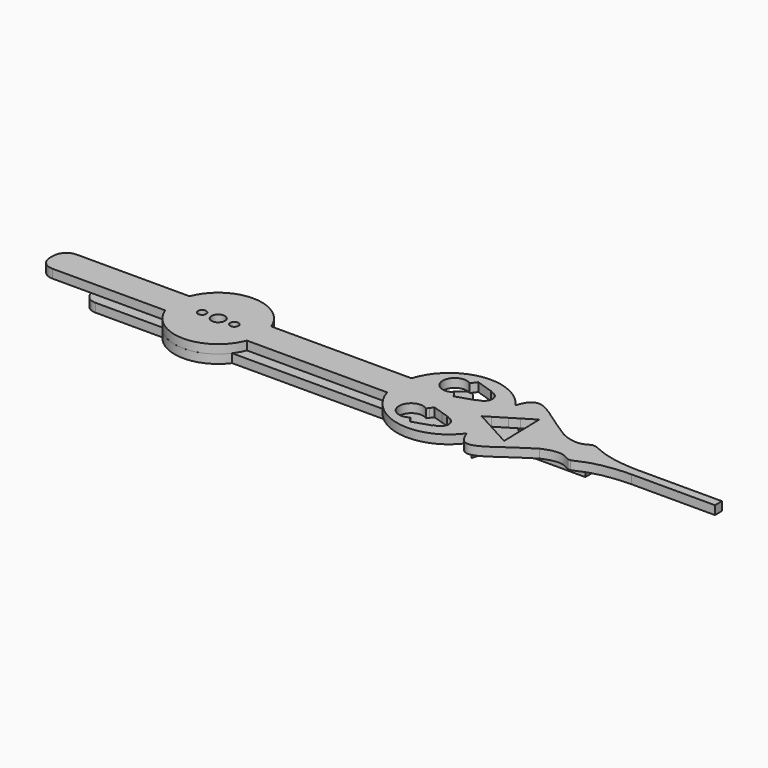
from build123d import *

# Parameters (mm, degrees)
F0_R     = 0.95
F0_R_2   = 1.5375
F1_DEPTH = 2
F2_R     = 0.95
F2_R_2   = 1.7859375
F3_DEPTH = 2
F4_R     = 3
F4_2_R   = 3


with BuildPart() as f1:
    # F0 (on Top) → F1 (new body)
    with BuildSketch(Plane.XY):
        with BuildLine():
            Line((-9.3674969976, 3.5), (-38.25, 3.5))
            Line((-38.25, 3.5), (-38.25, -3.5))
            Line((-38.25, -3.5), (-9.3674969976, -3.5))
            ThreePointArc((-9.3674969976, -3.5), (-10, 0), (-9.3674969976, 3.5))
        make_face()
        with BuildLine():
            ThreePointArc((9.3674969976, 3.5), (0, 10), (-9.3674969976, 3.5))
            Line((-9.3674969976, 3.5), (9.3674969976, 3.5))
        make_face()
        with BuildLine():
            Line((9.3674969976, 3.5), (-9.3674969976, 3.5))
            ThreePointArc((-9.3674969976, 3.5), (-10, 0), (-9.3674969976, -3.5))
            Line((-9.3674969976, -3.5), (9.3674969976, -3.5))
            ThreePointArc((9.3674969976, -3.5), (9.8406038935, -1.7783461452), (10, 0))
            ThreePointArc((10, 0), (9.8406038935, 1.7783461452), (9.3674969976, 3.5))
        make_face()
        with Locations((-3.7, 0)):
            Circle(F0_R, mode=Mode.SUBTRACT)
        Circle(F0_R_2, mode=Mode.SUBTRACT)
        with Locations((3.7, 0)):
            Circle(F0_R, mode=Mode.SUBTRACT)
        with BuildLine():
            Line((41.5486460336, 3.5), (9.3674969976, 3.5))
            ThreePointArc((9.3674969976, 3.5), (9.8406038935, 1.7783461452), (10, 0))
            ThreePointArc((10, 0), (9.8406038935, -1.7783461452), (9.3674969976, -3.5))
            Line((9.3674969976, -3.5), (41.5486460336, -3.5))
            ThreePointArc((41.5486460336, -3.5), (41.0242157381, 0), (41.5486460336, 3.5))
        make_face()
        with BuildLine():
            Line((9.3674969976, -3.5), (-9.3674969976, -3.5))
            ThreePointArc((-9.3674969976, -3.5), (0, -10), (9.3674969976, -3.5))
        make_face()
        with BuildLine():
            ThreePointArc((62.6500663761, 6.9867862956), (51.0189547822, 11.7817934467), (41.5486460336, 3.5))
            Line((41.5486460336, 3.5), (51.2676081814, 3.5))
            Line((51.2676081814, 3.5), (50.8795437488, 4.034124869))
            ThreePointArc((50.8795437488, 4.034124869), (46.4980966164, 6.2665836886), (50.8795437488, 8.4990425082))
            Line((50.8795437488, 8.4990425082), (51.8198733731, 9.7932952023))
            Line((51.8198733731, 9.7932952023), (55.9657714069, 8.4462112726))
            Line((55.9657714069, 8.4462112726), (55.9657714069, 8.2063436542))
            ThreePointArc((55.9657714069, 8.2063436542), (57.3373888325, 7.6382011141), (57.9055313725, 6.2665836886))
            ThreePointArc((57.9055313725, 6.2665836886), (57.3373888325, 4.894966263), (55.9657714069, 4.3268237229))
            Line((55.9657714069, 4.3268237229), (55.9657714069, 4.0869561045))
            Line((55.9657714069, 4.0869561045), (54.1593062669, 3.5))
            Line((54.1593062669, 3.5), (62.0300889952, 3.5))
            add(Edge.make_bspline(
                [(62.6500663761, 6.9867862956), (62.325026984, 5.9395183136), (62.1150441282, 4.7229315023), (62.0300889952, 3.5)],
                knots=[0.7171634713, 0.7171634713, 0.7171634713, 0.7171634713, 0.8591293722, 0.8591293722, 0.8591293722, 0.8591293722], degree=3))
        make_face()
        with BuildLine():
            Line((51.2676081814, 3.5), (41.5486460336, 3.5))
            ThreePointArc((41.5486460336, 3.5), (41.0242157381, 0), (41.5486460336, -3.5))
            Line((41.5486460336, -3.5), (51.2676081814, -3.5))
            Line((51.2676081814, -3.5), (51.8198733731, -2.7398721748))
            Line((51.8198733731, -2.7398721748), (54.1593062669, -3.5))
            Line((54.1593062669, -3.5), (62.0300889952, -3.5))
            add(Edge.make_bspline(
                [(62.0300889952, -3.5), (61.9699977026, -2.634984173), (61.9724597012, -1.7667939996), (62.0410036734, -0.953104062)],
                knots=[0.8591293722, 0.8591293722, 0.8591293722, 0.8591293722, 0.9595460766, 0.9595460766, 0.9595460766, 0.9595460766], degree=3))
            Line((62.0410036734, -0.953104062), (60.5553723025, -0.141462227))
            Line((60.5553723025, -0.141462227), (62.057291222, 0.7735505189))
            add(Edge.make_bspline(
                [(62.0300889952, 3.5), (61.9655550988, 2.5710327675), (61.9731656392, 1.6384044737), (62.057291222, 0.7735505189)],
                knots=[0.8591293722, 0.8591293722, 0.8591293722, 0.8591293722, 0.9669699747, 0.9669699747, 0.9669699747, 0.9669699747], degree=3))
            Line((62.0300889952, 3.5), (54.1593062669, 3.5))
            Line((54.1593062669, 3.5), (51.8198733731, 2.7398721748))
            Line((51.8198733731, 2.7398721748), (51.2676081814, 3.5))
        make_face()
        with BuildLine():
            ThreePointArc((64.3828967802, 3.5), (63.6595501958, 5.3144940497), (62.6500663761, 6.9867862956))
            add(Edge.make_bspline(
                [(62.6500663761, 6.9867862956), (62.325026984, 5.9395183136), (62.1150441282, 4.7229315023), (62.0300889952, 3.5)],
                knots=[0.7171634713, 0.7171634713, 0.7171634713, 0.7171634713, 0.8591293722, 0.8591293722, 0.8591293722, 0.8591293722], degree=3))
            Line((62.0300889952, 3.5), (64.3828967802, 3.5))
        make_face()
        with BuildLine():
            add(Edge.make_bspline(
                [(76.5, 3.5), (70.4279765487, 7.1543273516), (65.4370003335, 12.5197019264), (63.0607100626, 8.3098689603), (62.6500663761, 6.9867862956)],
                knots=[0, 0, 0, 0, 0.5378085921, 0.7171634713, 0.7171634713, 0.7171634713, 0.7171634713], degree=3))
            ThreePointArc((62.6500663761, 6.9867862956), (63.6595501958, 5.3144940497), (64.3828967802, 3.5))
            Line((64.3828967802, 3.5), (66.5325360501, 3.5))
            Line((66.5325360501, 3.5), (69.4303606274, 5.2654391254))
            Line((69.4303606274, 5.2654391254), (69.4719960261, 3.5))
            Line((69.4719960261, 3.5), (76.5, 3.5))
        make_face()
        with BuildLine():
            Line((51.2676081814, -3.5), (41.5486460336, -3.5))
            ThreePointArc((41.5486460336, -3.5), (51.0189547822, -11.7817934467), (62.6500663761, -6.9867862956))
            add(Edge.make_bspline(
                [(62.6500663761, -6.9867862956), (62.325026984, -5.9395183136), (62.1150441282, -4.7229315023), (62.0300889952, -3.5)],
                knots=[0.7171634713, 0.7171634713, 0.7171634713, 0.7171634713, 0.8591293722, 0.8591293722, 0.8591293722, 0.8591293722], degree=3))
            Line((62.0300889952, -3.5), (54.1593062669, -3.5))
            Line((54.1593062669, -3.5), (55.9657714069, -4.0869561045))
            Line((55.9657714069, -4.0869561045), (55.9657714069, -4.3268237229))
            ThreePointArc((55.9657714069, -4.3268237229), (57.3373888325, -4.894966263), (57.9055313725, -6.2665836886))
            ThreePointArc((57.9055313725, -6.2665836886), (57.3373888325, -7.6382011141), (55.9657714069, -8.2063436542))
            Line((55.9657714069, -8.2063436542), (55.9657714069, -8.4462112726))
            Line((55.9657714069, -8.4462112726), (51.8198733731, -9.7932952023))
            Line((51.8198733731, -9.7932952023), (50.8795437488, -8.4990425082))
            ThreePointArc((50.8795437488, -8.4990425082), (46.4980966164, -6.2665836886), (50.8795437488, -4.034124869))
            Line((50.8795437488, -4.034124869), (51.2676081814, -3.5))
        make_face()
        with BuildLine():
            add(Edge.make_bspline(
                [(76.5, 3.5), (81.0400280542, 1.4763858349), (82.0312268078, 3.2624417994), (83.0919519067, 3.5)],
                knots=[0, 0, 0, 0, 0.4179938527, 0.4179938527, 0.4179938527, 0.4179938527], degree=3))
            Line((76.5, 3.5), (69.4719960261, 3.5))
            Line((69.4719960261, 3.5), (69.6370811808, -3.5))
            Line((69.6370811808, -3.5), (76.5, -3.5))
            add(Edge.make_bspline(
                [(76.5, -3.5), (81.0400280542, -1.4763858349), (82.0312268078, -3.2624417994), (83.0919519067, -3.5)],
                knots=[0, 0, 0, 0, 0.4179938527, 0.4179938527, 0.4179938527, 0.4179938527], degree=3))
            Line((83.0919519067, -3.5), (83.6370610277, -3.5))
            add(Edge.make_bspline(
                [(83.6370610277, -3.5), (85.0624976542, -3.2313997522), (87.3028287907, -1.1404920716), (95.625, -1)],
                knots=[0.4871501593, 0.4871501593, 0.4871501593, 0.4871501593, 1, 1, 1, 1], degree=3))
            Line((95.625, -1), (114.75, -1))
            Line((114.75, -1), (114.75, 1))
            Line((114.75, 1), (95.625, 1))
            add(Edge.make_bspline(
                [(83.6370610277, 3.5), (85.0624976542, 3.2313997522), (87.3028287907, 1.1404920716), (95.625, 1)],
                knots=[0.4871501593, 0.4871501593, 0.4871501593, 0.4871501593, 1, 1, 1, 1], degree=3))
            Line((83.6370610277, 3.5), (83.0919519067, 3.5))
        make_face()
        with BuildLine():
            Line((64.3828967802, 3.5), (62.0300889952, 3.5))
            add(Edge.make_bspline(
                [(62.0300889952, 3.5), (61.9655550988, 2.5710327675), (61.9731656392, 1.6384044737), (62.057291222, 0.7735505189)],
                knots=[0.8591293722, 0.8591293722, 0.8591293722, 0.8591293722, 0.9669699747, 0.9669699747, 0.9669699747, 0.9669699747], degree=3))
            Line((62.057291222, 0.7735505189), (64.6706539693, 2.3656872131))
            ThreePointArc((64.6706539693, 2.3656872131), (64.5406787119, 2.936370663), (64.3828967802, 3.5))
        make_face()
        with BuildLine():
            Line((66.5325360501, 3.5), (64.3828967802, 3.5))
            ThreePointArc((64.3828967802, 3.5), (64.5406787119, 2.936370663), (64.6706539693, 2.3656872131))
            Line((64.6706539693, 2.3656872131), (66.5325360501, 3.5))
        make_face()
        with BuildLine():
            ThreePointArc((64.3828967802, -3.5), (63.6595501958, -5.3144940497), (62.6500663761, -6.9867862956))
            add(Edge.make_bspline(
                [(76.5, -3.5), (70.4279765487, -7.1543273516), (65.4370003335, -12.5197019264), (63.0607100626, -8.3098689603), (62.6500663761, -6.9867862956)],
                knots=[0, 0, 0, 0, 0.5378085921, 0.7171634713, 0.7171634713, 0.7171634713, 0.7171634713], degree=3))
            Line((76.5, -3.5), (69.6370811808, -3.5))
            Line((69.6370811808, -3.5), (69.6753803918, -5.1239768984))
            Line((69.6753803918, -5.1239768984), (66.7028487634, -3.5))
            Line((66.7028487634, -3.5), (64.3828967802, -3.5))
        make_face()
        with BuildLine():
            add(Edge.make_bspline(
                [(62.6500663761, -6.9867862956), (62.325026984, -5.9395183136), (62.1150441282, -4.7229315023), (62.0300889952, -3.5)],
                knots=[0.7171634713, 0.7171634713, 0.7171634713, 0.7171634713, 0.8591293722, 0.8591293722, 0.8591293722, 0.8591293722], degree=3))
            ThreePointArc((62.6500663761, -6.9867862956), (63.6595501958, -5.3144940497), (64.3828967802, -3.5))
            Line((64.3828967802, -3.5), (62.0300889952, -3.5))
        make_face()
        with BuildLine():
            add(Edge.make_bspline(
                [(62.0300889952, -3.5), (61.9699977026, -2.634984173), (61.9724597012, -1.7667939996), (62.0410036734, -0.953104062)],
                knots=[0.8591293722, 0.8591293722, 0.8591293722, 0.8591293722, 0.9595460766, 0.9595460766, 0.9595460766, 0.9595460766], degree=3))
            Line((62.0300889952, -3.5), (64.3828967802, -3.5))
            ThreePointArc((64.3828967802, -3.5), (64.5379557834, -2.9470833965), (64.6662544489, -2.3873517488))
            Line((64.6662544489, -2.3873517488), (62.0410036734, -0.953104062))
        make_face()
        with BuildLine():
            ThreePointArc((64.6662544489, -2.3873517488), (64.5379557834, -2.9470833965), (64.3828967802, -3.5))
            Line((64.3828967802, -3.5), (66.7028487634, -3.5))
            Line((66.7028487634, -3.5), (64.6662544489, -2.3873517488))
        make_face()
        with BuildLine():
            Line((83.6370610277, -3.5), (83.0919519067, -3.5))
            add(Edge.make_bspline(
                [(83.0919519067, -3.5), (83.2674469041, -3.5393035631), (83.4448450524, -3.5362199607), (83.6370610277, -3.5)],
                knots=[0.4179938527, 0.4179938527, 0.4179938527, 0.4179938527, 0.4871501593, 0.4871501593, 0.4871501593, 0.4871501593], degree=3))
        make_face()
    extrude(amount=F1_DEPTH)

    # F4
    f4_edges = [f1.edges().sort_by_distance(p)[0] for p in [
        (-38.25, 3.5, 1),
        (-38.25, -3.5, 1),
    ]]
    fillet(f4_edges, radius=F4_R)


with BuildPart() as f3:
    # F2 (on Top) → F3 (new body)
    with BuildSketch(Plane.XY):
        with BuildLine():
            Line((-8, 6), (-26.33333333, 6))
            Line((-26.33333333, 6), (-26.33333333, -6))
            Line((-26.33333333, -6), (-8, -6))
            ThreePointArc((-8, -6), (-10, 0), (-8, 6))
        make_face()
        with BuildLine():
            ThreePointArc((8, 6), (0, 10), (-8, 6))
            Line((-8, 6), (8, 6))
        make_face()
        with BuildLine():
            Line((8, -6), (-8, -6))
            ThreePointArc((-8, -6), (0, -10), (8, -6))
        make_face()
        with BuildLine():
            Line((53.6581738244, 6), (47.4167542526, 6))
            add(Edge.make_bspline(
                [(47.4167542526, 6), (46.3220957553, 4.3280086445), (45.5684344657, 2.1206918096), (46.0416666667, 0)],
                knots=[0.726906329, 0.726906329, 0.726906329, 0.726906329, 1, 1, 1, 1], degree=3))
            add(Edge.make_bspline(
                [(47.4167542526, -6), (46.3220957553, -4.3280086445), (45.5684344657, -2.1206918096), (46.0416666667, 0)],
                knots=[0.726906329, 0.726906329, 0.726906329, 0.726906329, 1, 1, 1, 1], degree=3))
            Line((47.4167542526, -6), (53.6581738244, -6))
            add(Edge.make_bspline(
                [(56.6666666667, -3.747044364), (55.2992674084, -4.4409490289), (54.3604326541, -5.2428049781), (53.6581738244, -6)],
                knots=[0, 0, 0, 0, 0.1542850544, 0.1542850544, 0.1542850544, 0.1542850544], degree=3))
            add(Edge.make_bspline(
                [(56.6666666667, -3.747044364), (60.0829150948, -2.2243293877), (62.0682583427, -4.2822499198), (63.2057347542, -6)],
                knots=[0, 0, 0, 0, 0.314529079, 0.314529079, 0.314529079, 0.314529079], degree=3))
            Line((63.2057347542, -6), (64.9547362718, -6))
            add(Edge.make_bspline(
                [(64.9547362718, -6), (65.4379538782, -4.0786939052), (66.6534703528, -1.3308020565), (70.8333333333, -1)],
                knots=[0.6769348689, 0.6769348689, 0.6769348689, 0.6769348689, 1, 1, 1, 1], degree=3))
            Line((70.8333333333, -1), (85, -1))
            Line((85, -1), (85, 1))
            Line((85, 1), (70.8333333333, 1))
            add(Edge.make_bspline(
                [(64.9547362718, 6), (65.4379538782, 4.0786939052), (66.6534703528, 1.3308020565), (70.8333333333, 1)],
                knots=[0.6769348689, 0.6769348689, 0.6769348689, 0.6769348689, 1, 1, 1, 1], degree=3))
            Line((64.9547362718, 6), (63.2057347542, 6))
            add(Edge.make_bspline(
                [(56.6666666667, 3.747044364), (60.0829150948, 2.2243293877), (62.0682583427, 4.2822499198), (63.2057347542, 6)],
                knots=[0, 0, 0, 0, 0.314529079, 0.314529079, 0.314529079, 0.314529079], degree=3))
            add(Edge.make_bspline(
                [(56.6666666667, 3.747044364), (55.2992674084, 4.4409490289), (54.3604326541, 5.2428049781), (53.6581738244, 6)],
                knots=[0, 0, 0, 0, 0.1542850544, 0.1542850544, 0.1542850544, 0.1542850544], degree=3))
        make_face()
        with BuildLine():
            Line((47.4167542526, 6), (8, 6))
            ThreePointArc((8, 6), (9.4868329805, 3.1622776602), (10, 0))
            ThreePointArc((10, 0), (9.4868329805, -3.1622776602), (8, -6))
            Line((8, -6), (47.4167542526, -6))
            add(Edge.make_bspline(
                [(47.4167542526, -6), (46.3220957553, -4.3280086445), (45.5684344657, -2.1206918096), (46.0416666667, 0)],
                knots=[0.726906329, 0.726906329, 0.726906329, 0.726906329, 1, 1, 1, 1], degree=3))
            add(Edge.make_bspline(
                [(47.4167542526, 6), (46.3220957553, 4.3280086445), (45.5684344657, 2.1206918096), (46.0416666667, 0)],
                knots=[0.726906329, 0.726906329, 0.726906329, 0.726906329, 1, 1, 1, 1], degree=3))
        make_face()
        with BuildLine():
            Line((8, 6), (-8, 6))
            ThreePointArc((-8, 6), (-10, 0), (-8, -6))
            Line((-8, -6), (8, -6))
            ThreePointArc((8, -6), (9.4868329805, -3.1622776602), (10, 0))
            ThreePointArc((10, 0), (9.4868329805, 3.1622776602), (8, 6))
        make_face()
        with Locations((-3.7, 0)):
            Circle(F2_R, mode=Mode.SUBTRACT)
        Circle(F2_R_2, mode=Mode.SUBTRACT)
        with Locations((3.7, 0)):
            Circle(F2_R, mode=Mode.SUBTRACT)
        with BuildLine():
            Line((64.9547362718, -6), (63.2057347542, -6))
            add(Edge.make_bspline(
                [(63.2057347542, -6), (63.8460680348, -6.9669937179), (64.6067347392, -8.7255695183), (64.6775118095, -7.1022633325), (64.9547362718, -6)],
                knots=[0.314529079, 0.314529079, 0.314529079, 0.314529079, 0.4915907173, 0.6769348689, 0.6769348689, 0.6769348689, 0.6769348689], degree=3))
        make_face()
        with BuildLine():
            add(Edge.make_bspline(
                [(63.2057347542, 6), (63.8460680348, 6.9669937179), (64.6067347392, 8.7255695183), (64.6775118095, 7.1022633325), (64.9547362718, 6)],
                knots=[0.314529079, 0.314529079, 0.314529079, 0.314529079, 0.4915907173, 0.6769348689, 0.6769348689, 0.6769348689, 0.6769348689], degree=3))
            Line((63.2057347542, 6), (64.9547362718, 6))
        make_face()
        with BuildLine():
            add(Edge.make_bspline(
                [(53.6581738244, 6), (52.2194091826, 7.5513160935), (51.4119093355, 10.0220105563), (48.4450081755, 7.5705644038), (47.4167542526, 6)],
                knots=[0.1542850544, 0.1542850544, 0.1542850544, 0.1542850544, 0.4703791662, 0.726906329, 0.726906329, 0.726906329, 0.726906329], degree=3))
            Line((47.4167542526, 6), (53.6581738244, 6))
        make_face()
        with BuildLine():
            Line((53.6581738244, -6), (47.4167542526, -6))
            add(Edge.make_bspline(
                [(53.6581738244, -6), (52.2194091826, -7.5513160935), (51.4119093355, -10.0220105563), (48.4450081755, -7.5705644038), (47.4167542526, -6)],
                knots=[0.1542850544, 0.1542850544, 0.1542850544, 0.1542850544, 0.4703791662, 0.726906329, 0.726906329, 0.726906329, 0.726906329], degree=3))
        make_face()
    extrude(amount=-F3_DEPTH)

    # F4#2
    f4_2_edges = [f3.edges().sort_by_distance(p)[0] for p in [
        (-26.333333, 6, -1),
        (-26.333333, -6, -1),
    ]]
    fillet(f4_2_edges, radius=F4_2_R)


solid = Compound([f1.part, f3.part])
